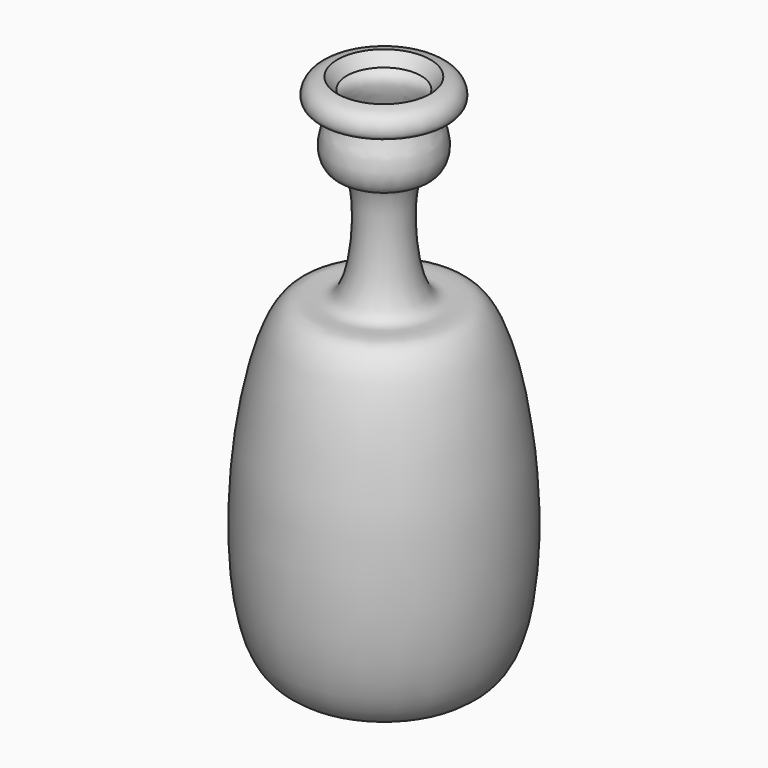
from build123d import *


with BuildPart() as f1:
    # F0 (on Front) → F1 (revolve)
    with BuildSketch(Plane.XZ):
        with BuildLine():
            Line((-10.3818709818, 69.357964862), (-13.0017824279, 72.493664603))
            add(Edge.make_bspline(
                [(-13.0017824279, 72.493664603), (-14.668265092, 72.3567175425), (-18.2998713612, 71.2146510263), (-19.011657494, 64.3052474439), (-9.220600462, 67.3558520782), (-16.2144642275, 57.3702098399), (-12.7715770094, 48.7394604501), (-5.5547802993, 51.6103408405), (-7.0624392322, 10.1774762065), (-30.5274444983, 28.8672071439), (-42.6249115932, -84.1043662647), (-11.5204223575, -76.4801217827), (0, -73.6562684178)],
                knots=[0.0699289622, 0.0699289622, 0.0699289622, 0.0699289622, 0.1036053802, 0.1596824081, 0.2172140524, 0.2896222141, 0.3593047578, 0.4089791655, 0.5468784547, 0.6315136623, 0.8635207217, 1, 1, 1, 1], degree=3))
            Line((0, -73.6562684178), (0, -70.126414299))
            add(Edge.make_bspline(
                [(-10.3818709818, 69.357964862), (-12.6563804505, 69.6243971803), (-16.8567539167, 70.0306970134), (-8.7823589785, 68.0988594592), (-11.0412079697, 61.0593928897), (-13.0468385533, 55.8451267698), (-3.8075104954, 50.2781858052), (-6.761750988, 23.2849340676), (-8.5498645502, 14.5229346594), (-26.9722051735, 20.4818981963), (-34.6250310629, -41.8781800996), (-28.1512531426, -69.1552864555), (-19.6761033053, -75.3646023556), (-4.5873783925, -72.7420548139), (-1.2488761645, -70.8385009887), (0, -70.126414299)],
                knots=[0.0742592578, 0.0742592578, 0.0742592578, 0.0742592578, 0.1128224182, 0.1560958562, 0.2085940577, 0.2540137873, 0.3146427544, 0.4220053608, 0.4768912445, 0.5445759059, 0.7007399959, 0.8129149903, 0.8735606391, 0.9527012135, 1, 1, 1, 1], degree=3))
        make_face()
    revolve(axis=Axis((0, 0, -73.6562646925), (0, 0, -1)))


solid = f1.part
